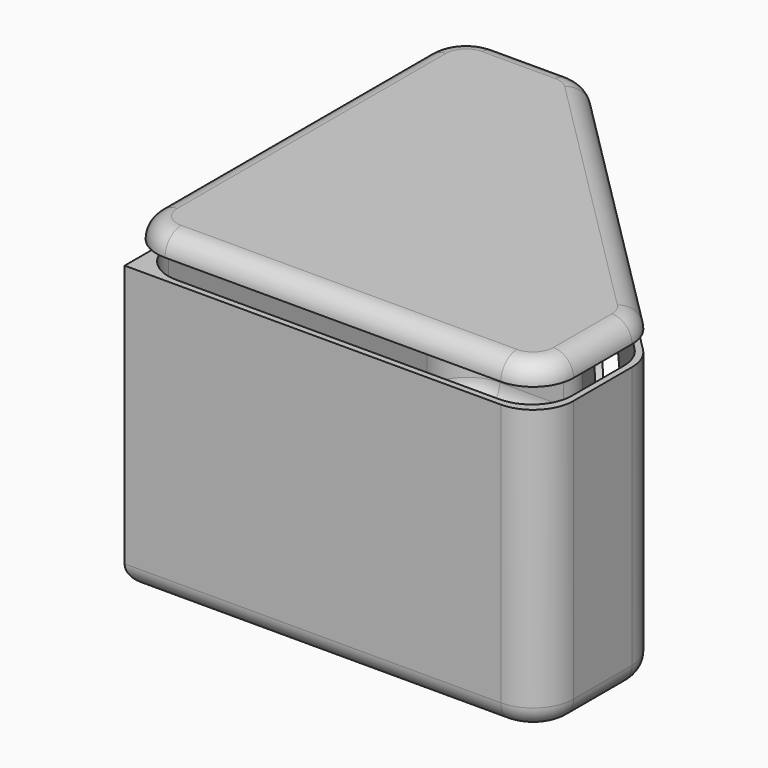
from build123d import *

# Parameters (mm, degrees)
F3_DEPTH = 6.35
F4_DEPTH = 88.9
F5_DEPTH = 2.54
F6_R     = 31.9402199722
F7_DEPTH = 25.4
F8_R     = 12.7
F9_R     = 12.7
F10_R    = 6.34999
F11_R    = 6.35


# Not quite as in the source:
# - a fillet or chamfer is up to 0.001 mm smaller than in the source, because OpenCascade refuses the exact size


with BuildPart() as f3:
    # F2 (on offset) → F3 (new body)
    with BuildSketch(Plane.XY.offset(101.6)):
        Polygon((-129.0066, 2.0066), (-2.0066, 2.0066), (-2.0066, 40.1066), (-90.9066, 129.0066), (-129.0066, 129.0066), align=None)
        Polygon((-2.0066, 2.0066), (0, 0), (0, 40.9377609343), (-2.0066, 40.1066), align=None)
        Polygon((-90.0754390657, 131.0132), (-131.0132, 131.0132), (-129.0066, 129.0066), (-90.9066, 129.0066), align=None)
        Polygon((-2.0066, 40.1066), (0, 40.9377609343), (-90.0754390657, 131.0132), (-90.9066, 129.0066), align=None)
        Polygon((-131.0132, 0), (0, 0), (-2.0066, 2.0066), (-129.0066, 2.0066), align=None)
        Polygon((-131.0132, 131.0132), (-131.0132, 0), (-129.0066, 2.0066), (-129.0066, 129.0066), align=None)
    extrude(amount=-F3_DEPTH)

    # F9
    f9_edges = [f3.edges().sort_by_distance(p)[0] for p in [
        (0, 40.937761, 98.425),
        (-90.075439, 131.0132, 98.425),
        (-131.0132, 131.0132, 98.425),
        (-131.0132, 0, 98.425),
        (0, 0, 98.425),
    ]]
    fillet(f9_edges, radius=F9_R)

    # F10 (radius 6.35 in the source; OpenCascade refuses exactly that, so slightly less here)
    f10_edges = [f3.edges().sort_by_distance(p)[0] for p in [
        (0, 24.188624, 101.6),
        (-3.719744, 3.719744, 101.6),
        (-0.96673, 40.537328, 101.6),
        (-65.5066, 0, 101.6),
        (-45.03772, 85.97548, 101.6),
        (-127.293456, 3.719744, 101.6),
        (-90.475872, 130.04647, 101.6),
        (-131.0132, 65.5066, 101.6),
        (-106.824576, 131.0132, 101.6),
        (-127.293456, 127.293456, 101.6),
    ]]
    fillet(f10_edges, radius=F10_R)


with BuildPart() as f4:
    # F0 (on Top) → F4 (new body)
    with BuildSketch(Plane.XY):
        Polygon((-90.0715728753, 131), (-131, 131), (-131, 0), (0, 0), (0, 40.9284271247), align=None)
        Polygon((-129, 2), (-129, 129), (-90.9, 129), (-2, 40.1), (-2, 2), align=None, mode=Mode.SUBTRACT)
    extrude(amount=F4_DEPTH)

    # F0 (on Top) → F5 (join)
    with BuildSketch(Plane.XY):
        Polygon((-90.9, 129), (-129, 129), (-129, 2), (-2, 2), (-2, 40.1), align=None)
    extrude(amount=F5_DEPTH)

    # F6 (on face) → F7 (cut)
    with BuildSketch(Plane(origin=(20.4642135624, 20.4642135624, 0), x_dir=(-0.7071067812, 0.7071067812, 0), z_dir=(0.7071067812, 0.7071067812, 0))):
        with Locations((92.6309883354, 44.6402199722)):
            Circle(F6_R)
    extrude(amount=-F7_DEPTH, mode=Mode.SUBTRACT)

    # F8
    f8_edges = [f4.edges().sort_by_distance(p)[0] for p in [
        (0, 40.928427, 44.45),
        (0, 0, 44.45),
        (-90.071573, 131, 44.45),
        (-131, 131, 44.45),
        (-129, 2, 45.72),
        (-2, 2, 45.72),
        (-2, 40.1, 45.72),
        (-90.9, 129, 45.72),
        (-129, 129, 45.72),
    ]]
    fillet(f8_edges, radius=F8_R)

    # F11
    f11_edges = [f4.edges().sort_by_distance(p)[0] for p in [
        (-106.230256, 129, 2.54),
        (-91.300433, 128.03327, 2.54),
        (-125.280256, 125.280256, 2.54),
        (-46.45, 84.55, 2.54),
        (-129, 65.5, 2.54),
        (-2.96673, 39.699567, 2.54),
        (-125.280256, 5.719744, 2.54),
        (-2, 24.769744, 2.54),
        (-65.5, 2, 2.54),
        (-5.719744, 5.719744, 2.54),
        (-45.035786, 85.964214, 0),
        (-0.96673, 40.527994, 0),
        (-90.472006, 130.03327, 0),
        (0, 24.183957, 0),
        (-106.816043, 131, 0),
        (-3.719744, 3.719744, 0),
        (-127.280256, 127.280256, 0),
        (-71.85, 0, 0),
        (-131, 59.15, 0),
    ]]
    fillet(f11_edges, radius=F11_R)


solid = Compound([f3.part, f4.part])
